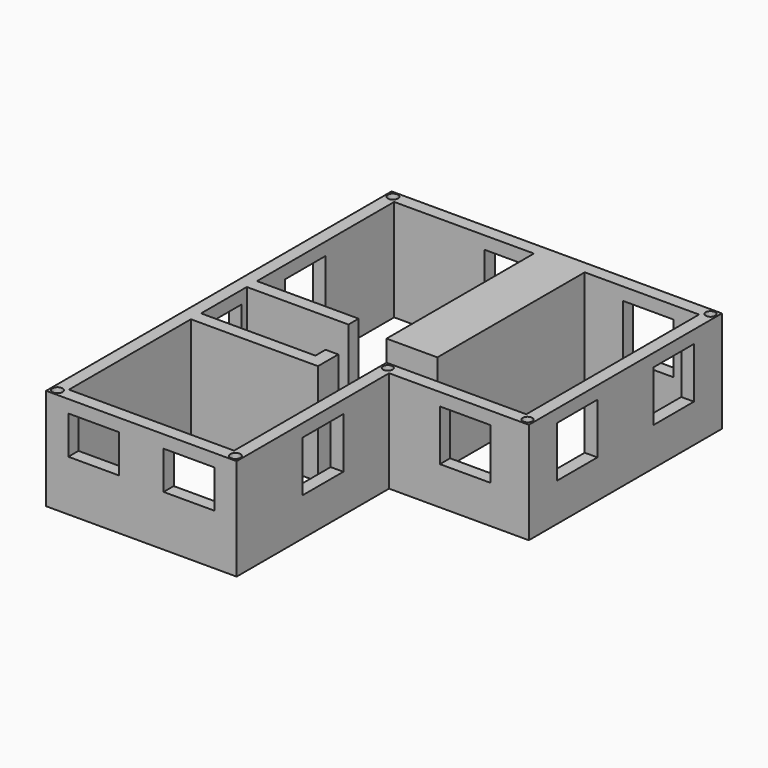
from build123d import *

# Parameters (mm, degrees)
F0_W      = 101.6
F0_H      = 368.3
F0_W_2    = 203.2
F0_H_2    = 25.4
F1_DEPTH  = 203.2
F2_R      = 10.16
F2_R_2    = 9.525
F3_DEPTH  = 12.7
F4_DEPTH  = 203.2
F5_DEPTH  = 31.75
F6_W      = 50.8
F6_H      = 76.2
F7_DEPTH  = 25.4
F9_DEPTH  = 25.4
F11_DEPTH = 2540
F13_DEPTH = 25.4
F15_DEPTH = 25.4
F16_W     = 88.9
F16_H     = 76.2
F17_DEPTH = 25.4
F16_W_2   = 101.6
F16_H_2   = 101.6
F18_DEPTH = 25.4
F19_R     = 9.525
F20_DEPTH = 19.05


# Not quite as in the source:
# - a feature names something its author has since deleted; it is built from what else it names


with BuildPart() as f1:
    # F0 (on Top) → F1 (new body)
    with BuildSketch(Plane.XY):
        Polygon((0, 863.6), (0, 0), (381, 0), (381, 381), (660.4, 381), (660.4, 406.4), (660.4, 838.2), (660.4, 863.6), align=None)
        Polygon((406.4, 838.2), (635, 838.2), (635, 406.4), (355.6, 406.4), (355.6, 25.4), (25.4, 25.4), (25.4, 38.7719720602), (25.4, 330.2), (25.4, 355.6), (25.4, 469.9), (25.4, 495.3), (25.4, 838.2), (304.8, 838.2), align=None, mode=Mode.SUBTRACT)
        with Locations((355.6, 654.05)):
            Rectangle(F0_W, F0_H)
        Polygon((254, 355.6), (25.4, 355.6), (25.4, 330.2), (279.4, 330.2), (279.4, 355.6), (279.4, 381), (254, 381), align=None)
        with Locations((127, 482.6)):
            Rectangle(F0_W_2, F0_H_2)
    extrude(amount=F1_DEPTH)

    # F2 (on face) → F3 (cut)
    with BuildSketch(Plane(origin=(0, 0, 0), x_dir=(1, 0, 0), z_dir=(0, 0, -1))):
        with Locations((12.7, -850.9)):
            Circle(F2_R)
        with Locations((12.7, -12.7)):
            Circle(F2_R)
        with Locations((368.3, -12.7)):
            Circle(F2_R)
        with Locations((647.7, -850.9)):
            Circle(F2_R_2)
        with Locations((368.3, -393.7)):
            Circle(F2_R_2)
        with Locations((647.7, -393.7)):
            Circle(F2_R_2)
    extrude(amount=-F3_DEPTH, mode=Mode.SUBTRACT)

    # F4 (add): faces of the model
    f4_faces = [f1.faces().sort_by_distance(p)[0] for p in [
        (12.7, 12.7, 12.7),
        (368.3, 12.7, 12.7),
        (12.7, 850.9, 12.7),
    ]]
    extrude(f4_faces, amount=-F4_DEPTH)

    # F5 (cut): faces of the model
    f5_faces = [f1.faces().sort_by_distance(p)[0] for p in [
        (12.7, 850.9, 215.9),
        (368.3, 12.7, 215.9),
        (12.7, 12.7, 215.9),
    ]]
    extrude(f5_faces, amount=-F5_DEPTH, mode=Mode.SUBTRACT)

    # F6 (on face) → F7 (cut)
    with BuildSketch(Plane.XZ):
        with Locations((120.65, 139.7)):
            Rectangle(F6_W, F6_H)
        with Locations((69.85, 139.7)):
            Rectangle(F6_W, F6_H)
        Polygon((234.95, 177.8), (234.95, 101.6), (336.55, 101.6), (336.55, 177.8), (285.75, 177.8), align=None)
    extrude(amount=-F7_DEPTH, mode=Mode.SUBTRACT)

    # F8 (on face) → F9 (cut)
    with BuildSketch(Plane.YZ.offset(381)):
        Polygon((165.1, 76.2), (190.5, 76.2), (266.7, 76.2), (266.7, 177.8), (165.1, 177.8), align=None)
    extrude(amount=-F9_DEPTH, mode=Mode.SUBTRACT)

    # F10 (on face) → F11 (cut)
    with BuildSketch(Plane.XZ.offset(-381)):
        Polygon((482.6, 76.2), (533.4, 76.2), (584.2, 76.2), (584.2, 177.8), (482.6, 177.8), align=None)
    extrude(amount=-F11_DEPTH, mode=Mode.SUBTRACT)

    # F12 (on face) → F13 (cut)
    with BuildSketch(Plane.YZ.offset(660.4)):
        Polygon((450.85, 76.2), (501.65, 76.2), (552.45, 76.2), (552.45, 177.8), (450.85, 177.8), align=None)
        Polygon((793.75, 177.8), (692.15, 177.8), (692.15, 76.2), (742.95, 76.2), (793.75, 76.2), align=None)
    extrude(amount=-F13_DEPTH, mode=Mode.SUBTRACT)

    # F14 (on face) → F15 (cut)
    with BuildSketch(Plane(origin=(0, 863.6, 0), x_dir=(-1, 0, 0), z_dir=(0, 1, 0))):
        Polygon((-206.375, 177.8), (-257.175, 177.8), (-307.975, 177.8), (-307.975, 76.2), (-206.375, 76.2), align=None)
    extrude(amount=-F15_DEPTH, mode=Mode.SUBTRACT)

    # F16 (on face) → F17 (cut)
    with BuildSketch(Plane(origin=(0, 0, 0), x_dir=(0, -1, 0), z_dir=(-1, 0, 0))):
        with Locations((-412.75, 139.7)):
            Rectangle(F16_W, F16_H)
    extrude(amount=-F17_DEPTH, mode=Mode.SUBTRACT)

    # F16 (on face) → F18 (cut)
    with BuildSketch(Plane(origin=(0, 0, 0), x_dir=(0, -1, 0), z_dir=(-1, 0, 0))):
        with Locations((-412.75, 139.7)):
            Rectangle(F16_W, F16_H)
        with Locations((-615.95, 127)):
            Rectangle(F16_W_2, F16_H_2)
    extrude(amount=-F18_DEPTH, mode=Mode.SUBTRACT)

    # F19 (on face) → F20 (cut)
    with BuildSketch(Plane.XY.offset(203.2)):
        with Locations((368.3, 393.7)):
            Circle(F19_R)
        with Locations((647.7, 393.7)):
            Circle(F19_R)
        with Locations((647.7, 850.9)):
            Circle(F19_R)
    extrude(amount=-F20_DEPTH, mode=Mode.SUBTRACT)


solid = f1.part
